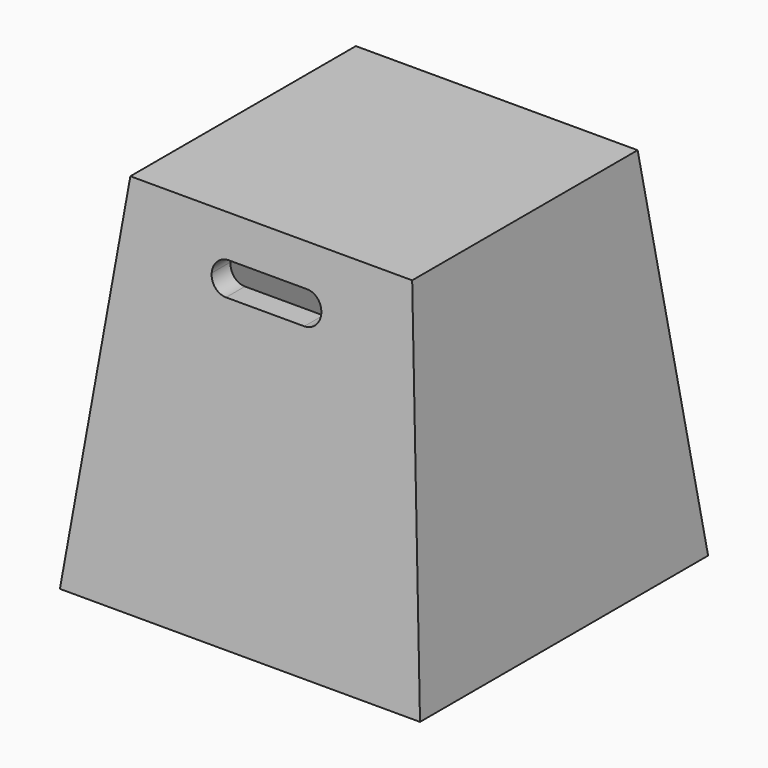
from build123d import *

# Parameters (mm, degrees)
F1_W          = 23
F1_H          = 23
F2_W          = 18
F2_H          = 18
F4_T          = -1.5
F5_W          = 7
F5_H          = 2
F6_DEPTH      = 11.5010001
F6_DEPTH_BACK = 11.5010001
F7_R          = 0.9999


# Not quite as in the source:
# - a fillet or chamfer is up to 0.001 mm smaller than in the source, because OpenCascade refuses the exact size


with BuildPart() as f3:
    # F1 (on Top) → F3 section 0
    with BuildSketch(Plane.XY):
        Rectangle(F1_W, F1_H)
    # F2 (on offset) → F3 section 1
    with BuildSketch(Plane.XY.offset(23)):
        Rectangle(F2_W, F2_H)
    loft()

    # F4
    f4_openings = [f3.faces().sort_by_distance(p)[0] for p in [
        (0, 0, 0),
    ]]
    offset(amount=F4_T, openings=f4_openings)

    # F5 (on Front) → F6 (cut, two sides)
    with BuildSketch(Plane.XZ) as f6_sk:
        with Locations((0, 19.5)):
            Rectangle(F5_W, F5_H)
    extrude(amount=-F6_DEPTH, mode=Mode.SUBTRACT)
    extrude(f6_sk.sketch, amount=F6_DEPTH_BACK, mode=Mode.SUBTRACT)

    # F7 (radius 1 in the source; OpenCascade refuses exactly that, so slightly less here)
    f7_edges = [f3.edges().sort_by_distance(p)[0] for p in [
        (-3.5, 8.517322, 20.5),
        (-3.5, -8.517322, 20.5),
        (-3.5, 8.734713, 18.5),
        (-3.5, -8.734713, 18.5),
        (3.5, 8.734713, 18.5),
        (3.5, -8.734713, 18.5),
        (3.5, 8.517322, 20.5),
        (3.5, -8.517322, 20.5),
    ]]
    fillet(f7_edges, radius=F7_R)


solid = f3.part
